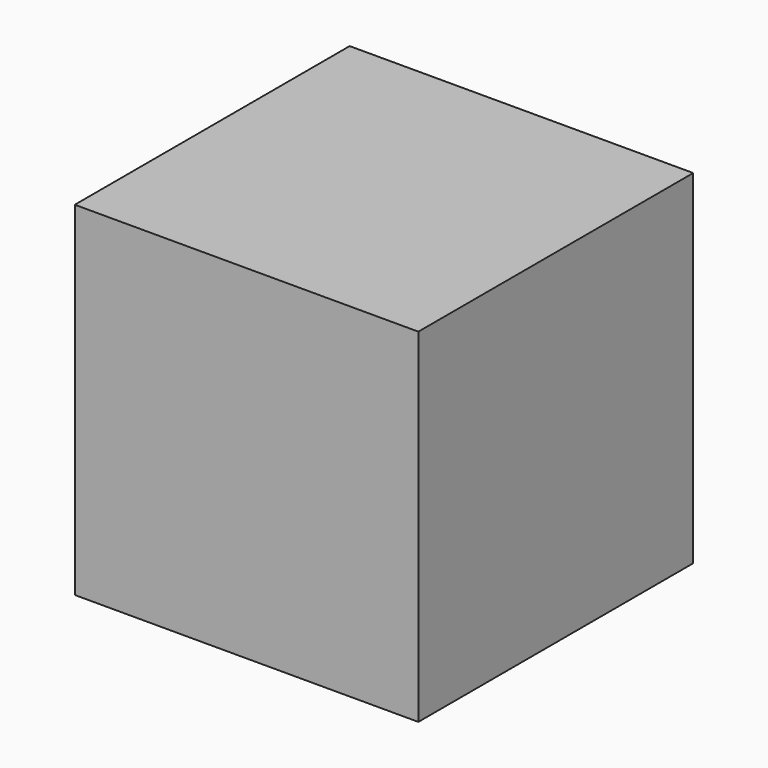
from build123d import *

# Parameters (mm, degrees)
F0_W     = 152.4
F0_H     = 152.4
F1_DEPTH = 152.4
F5_DEPTH = 50.8


# Not quite as in the source:
# - the program builds the solid bodies; features that only make, move or delete a surface that nothing else refers to are left out


with BuildPart() as f1:
    # F0 (on Top) → F1 (new body)
    with BuildSketch(Plane.XY):
        Rectangle(F0_W, F0_H)
    extrude(amount=F1_DEPTH)

    # F4 (on face) → F5 (cut)
    with BuildSketch(Plane(origin=(0, 76.2, 0), x_dir=(-1, 0, 0), z_dir=(0, 1, 0))):
        Polygon((-1.9910766715, 26.005651243), (36.5384817123, 45.9516048431), (38.5295583838, 89.2921580002), (1.9910766715, 112.6867575571), (-36.5384817123, 92.740803957), (-38.5295583838, 49.4002507999), align=None)
    extrude(amount=-F5_DEPTH, mode=Mode.SUBTRACT)


solid = f1.part
